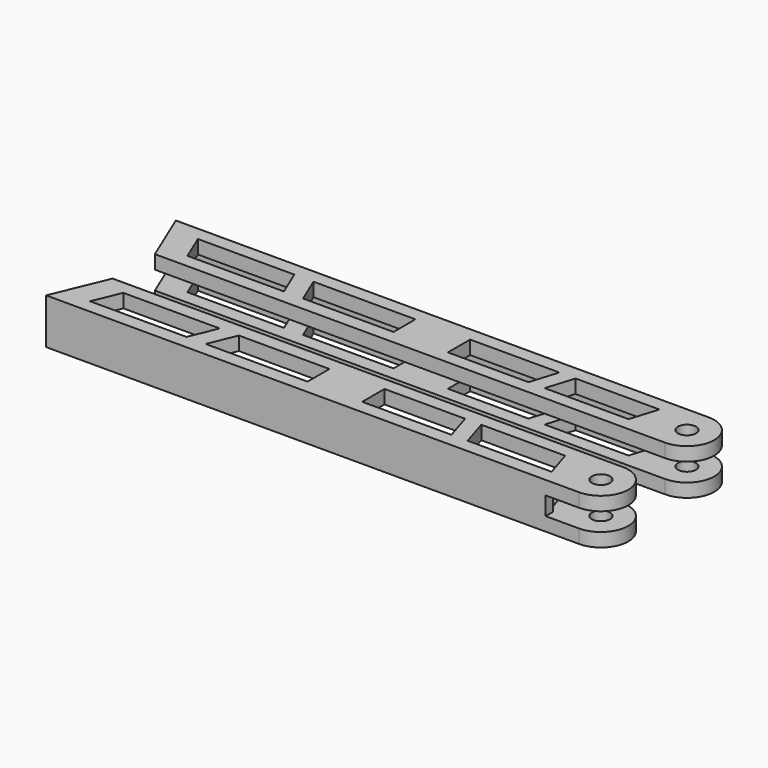
from build123d import *

# Parameters (mm, degrees)
F0_R      = 2
F1_DEPTH  = 10
F2_W      = 10.1941861212
F2_H      = 4.0345681068
F3_DEPTH  = 10
F4_W      = 7.5655020773
F4_H      = 4
F5_DEPTH  = 5
F6_W      = 11.8742840528
F6_H      = 0.0345681068
F7_DEPTH  = 5
F8_W      = 22.0980979502
F8_H      = 4
F9_DEPTH  = 10
F10_W     = 8.841574192
F10_H     = 4
F11_DEPTH = 5


with BuildPart() as f1:
    # F0 (on Top) → F1 (new body)
    with BuildSketch(Plane.XY):
        with BuildLine():
            Line((-73.2878747284, 5.7992432788), (38.7121252716, 5.7992432788))
            ThreePointArc((38.7121252716, 5.7992432788), (44.7121252716, 11.7992432788), (38.7121252716, 17.7992432788))
            Line((38.7121252716, 17.7992432788), (-78.2878747284, 17.7992432788))
            Line((-78.2878747284, 17.7992432788), (-73.2878747284, 5.7992432788))
        make_face()
        Polygon((-47.3650060594, 8.7992432788), (-68.5378747284, 8.7992432788), (-71.0378747284, 14.7992432788), (-49.8650060594, 14.7992432788), align=None, mode=Mode.SUBTRACT)
        Polygon((-45.6628747284, 14.7992432788), (-23.2878747284, 14.7992432788), (-23.2878747284, 8.7992432788), (-43.1628747284, 8.7992432788), align=None, mode=Mode.SUBTRACT)
        Polygon((-11.2878747284, 8.6967073874), (-11.2878747284, 14.7992432788), (8.3094434813, 14.7992432788), (6.401501639, 8.6967073874), align=None, mode=Mode.SUBTRACT)
        Polygon((9.9537555186, 8.6967073874), (11.8616973609, 14.7992432788), (30.2808774263, 14.7992432788), (28.372935584, 8.6967073874), align=None, mode=Mode.SUBTRACT)
        with Locations((38.7121252716, 11.7992432788)):
            Circle(F0_R, mode=Mode.SUBTRACT)
    extrude(amount=F1_DEPTH)

    # F2 (on face) → F3 (cut)
    with BuildSketch(Plane.XZ.offset(-5.7992432788)):
        Polygon((-73.2878747284, 2.9654318932), (-73.2878747284, 7), (-77.6094347239, 7), (-78.6499679089, 7), (-78.6499679089, 2.9654318932), align=None)
        Polygon((38.7121252716, 7), (-70.0548663735, 7), (-73.2878747284, 7), (-73.2878747284, 2.9654318932), (-72.7878747284, 2.9654318932), (38.7121252716, 2.9654318932), align=None)
        with Locations((43.8092183322, 4.9827159466)):
            Rectangle(F2_W, F2_H)
    extrude(amount=-F3_DEPTH, mode=Mode.SUBTRACT)

    # F4 (on face) → F5 (cut)
    with BuildSketch(Plane(origin=(0, 17.7992432788, 0), x_dir=(-1, 0, 0), z_dir=(0, 1, 0))):
        with Locations((-42.4948763102, 5)):
            Rectangle(F4_W, F4_H)
        Polygon((-31.3099771738, 3), (-31.3099771738, 7), (-35.9585285187, 7), (-38.7121252716, 7), (-38.7121252716, 3), (-36.1494868994, 3), align=None)
    extrude(amount=-F5_DEPTH, mode=Mode.SUBTRACT)

    # F6 (on face) → F7 (cut)
    with BuildSketch(Plane.XZ.offset(-15.7992432788)):
        with Locations((37.2471192002, 2.9827159466)):
            Rectangle(F6_W, F6_H)
    extrude(amount=-F7_DEPTH, mode=Mode.SUBTRACT)


with BuildPart() as f1b:
    # F0 (on Top) → F1, piece 2 (new body)
    with BuildSketch(Plane.XY):
        with BuildLine():
            Line((-73.2878747284, -5.7992432788), (-78.2878747284, -17.7992432788))
            Line((-78.2878747284, -17.7992432788), (38.7121252716, -17.7992432788))
            ThreePointArc((38.7121252716, -17.7992432788), (44.7121252716, -11.7992432788), (38.7121252716, -5.7992432788))
            Line((38.7121252716, -5.7992432788), (-73.2878747284, -5.7992432788))
        make_face()
        Polygon((-47.3650060594, -8.7992432788), (-49.8650060594, -14.7992432788), (-71.0378747284, -14.7992432788), (-68.5378747284, -8.7992432788), align=None, mode=Mode.SUBTRACT)
        Polygon((-23.2878747284, -14.7992432788), (-45.6628747284, -14.7992432788), (-43.1628747284, -8.7992432788), (-23.2878747284, -8.7992432788), align=None, mode=Mode.SUBTRACT)
        Polygon((8.3094434813, -14.7992432788), (-11.2878747284, -14.7992432788), (-11.2878747284, -8.6967073874), (6.401501639, -8.6967073874), align=None, mode=Mode.SUBTRACT)
        Polygon((9.9537555186, -8.6967073874), (28.372935584, -8.6967073874), (30.2808774263, -14.7992432788), (11.8616973609, -14.7992432788), align=None, mode=Mode.SUBTRACT)
        with Locations((38.7121252716, -11.7992432788)):
            Circle(F0_R, mode=Mode.SUBTRACT)
    extrude(amount=F1_DEPTH)

    # F8 (on face) → F9 (cut)
    with BuildSketch(Plane(origin=(0, -5.7992432788, 0), x_dir=(-1, 0, 0), z_dir=(0, 1, 0))):
        Polygon((73.2878747284, 7), (-36.4116951823, 7), (-38.7121252716, 7), (-38.7121252716, 3), (-35.589389503, 3), (73.2878747284, 3), align=None)
        with Locations((-49.7611742467, 5)):
            Rectangle(F8_W, F8_H)
        Polygon((86.4499881864, 7), (73.2878747284, 7), (73.2878747284, 3), (86.6957977414, 3), align=None)
    extrude(amount=-F9_DEPTH, mode=Mode.SUBTRACT)

    # F10 (on face) → F11 (cut)
    with BuildSketch(Plane.XZ.offset(17.7992432788)):
        Polygon((34.7536914051, 3), (38.7121252716, 3), (38.7121252716, 7), (34.7536914051, 7), (31.3738286495, 7), (31.3738286495, 3), align=None)
        with Locations((43.1329123676, 5)):
            Rectangle(F10_W, F10_H)
    extrude(amount=-F11_DEPTH, mode=Mode.SUBTRACT)


solid = Compound([f1.part, f1b.part])
